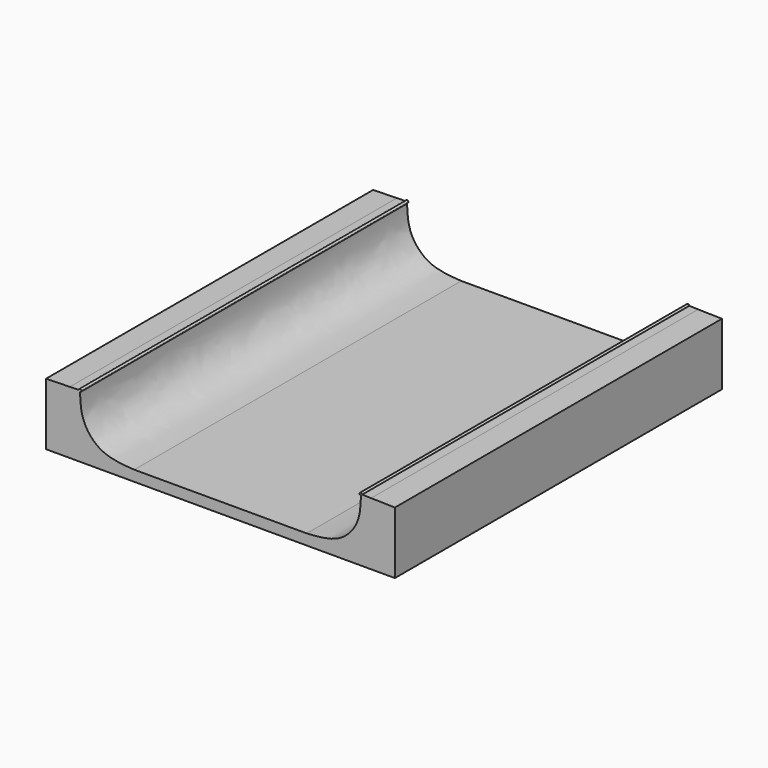
from build123d import *

# Parameters (mm, degrees)
F0_W     = 107.1716099977
F0_H     = 6.6367755644
F1_DEPTH = 254


# Not quite as in the source:
# - ends of sketch curves that miss each other by under 0.0002 mm in the source are joined


with BuildPart() as f1:
    # F0 (on Front) → F1 (new body)
    with BuildSketch(Plane.XZ):
        with BuildLine():
            Line((-53.5858049989, -3.3183877822), (-53.5858049989, 3.3183877822))
            add(Edge.make_bspline(
                [(-53.5858049989, 3.3183877822), (-60.7905189574, 3.7842082585), (-74.5629530695, 4.6746644037), (-86.6963968754, 19.2661575582), (-87.1229924092, 29.8680118762), (-87.2426380733, 34.9518884332)],
                knots=[0, 0, 0, 0, 0.3582791422, 0.6848815801, 0.984054993, 0.984054993, 0.984054993, 0.984054993], degree=3))
            ThreePointArc((-87.2426380733, 34.9518884332), (-87.8230310318, 35.1768908631), (-88.0742459033, 35.7464285425))
            Line((-88.0742459033, 35.7464285425), (-93.6096602081, 35.6210684855))
            Line((-93.6096602081, 35.6210684855), (-108.3679497242, 35.286838758))
            Line((-108.3679497242, 35.286838758), (-108.3679497242, -3.3183877822))
            Line((-108.3679497242, -3.3183877822), (-53.5858049989, -3.3183877822))
        make_face()
        with BuildLine():
            add(Edge.make_bspline(
                [(53.5858049989, 3.3183877822), (60.7905189574, 3.7842082585), (74.5629530695, 4.6746644037), (86.6963968754, 19.2661575582), (87.1229924092, 29.8680118762), (87.2426380733, 34.9518884332)],
                knots=[0, 0, 0, 0, 0.3582791422, 0.6848815801, 0.984054993, 0.984054993, 0.984054993, 0.984054993], degree=3))
            Line((53.5858049989, 3.3183877822), (53.5858049989, -3.3183877822))
            Line((53.5858049989, -3.3183877822), (108.3679497242, -3.3183877822))
            Line((108.3679497242, -3.3183877822), (108.3679497242, 35.286838758))
            Line((108.3679497242, 35.286838758), (93.6096602081, 35.6210684855))
            Line((93.6096602081, 35.6210684855), (88.0742459033, 35.7464285425))
            ThreePointArc((88.0742459033, 35.7464285425), (87.8230310318, 35.1768908631), (87.2426380733, 34.9518884332))
        make_face()
        Rectangle(F0_W, F0_H)
        with BuildLine():
            add(Edge.make_bspline(
                [(-87.2426380733, 34.9518884332), (-87.2490148129, 35.2228431489), (-87.2551520855, 35.4938413246), (-87.2612893581, 35.7648395002)],
                knots=[0.984054993, 0.984054993, 0.984054993, 0.984054993, 1, 1, 1, 1], degree=3))
            ThreePointArc((-87.2426380733, 34.9518884332), (-86.6797380364, 35.1964774959), (-86.448124364, 35.7648395002))
            ThreePointArc((-86.448124364, 35.7648395002), (-87.270495427, 36.5779523805), (-88.0742459033, 35.7464285425))
            Line((-88.0742459033, 35.7464285425), (-87.2612893581, 35.7648395002))
        make_face()
        with BuildLine():
            ThreePointArc((-88.0742459033, 35.7464285425), (-87.8230310318, 35.1768908631), (-87.2426380733, 34.9518884332))
            add(Edge.make_bspline(
                [(-87.2426380733, 34.9518884332), (-87.2490148129, 35.2228431489), (-87.2551520855, 35.4938413246), (-87.2612893581, 35.7648395002)],
                knots=[0.984054993, 0.984054993, 0.984054993, 0.984054993, 1, 1, 1, 1], degree=3))
            Line((-87.2612893581, 35.7648395002), (-88.0742459033, 35.7464285425))
        make_face()
        with BuildLine():
            add(Edge.make_bspline(
                [(87.2426380733, 34.9518884332), (87.2490148129, 35.2228431489), (87.2551520855, 35.4938413246), (87.2612893581, 35.7648395002)],
                knots=[0.984054993, 0.984054993, 0.984054993, 0.984054993, 1, 1, 1, 1], degree=3))
            ThreePointArc((87.2426380733, 34.9518884332), (87.8230310318, 35.1768908631), (88.0742459033, 35.7464285425))
            Line((88.0742459033, 35.7464285425), (87.2612893581, 35.7648395002))
        make_face()
        with BuildLine():
            ThreePointArc((88.0744543523, 35.7648395002), (86.6929273539, 36.346390822), (87.2426380733, 34.9518884332))
            add(Edge.make_bspline(
                [(87.2426380733, 34.9518884332), (87.2490148129, 35.2228431489), (87.2551520855, 35.4938413246), (87.2612893581, 35.7648395002)],
                knots=[0.984054993, 0.984054993, 0.984054993, 0.984054993, 1, 1, 1, 1], degree=3))
            Line((87.2612893581, 35.7648395002), (88.0742459033, 35.7464285425))
            ThreePointArc((88.0742459033, 35.7464285425), (88.0744022384, 35.7556334313), (88.0744543523, 35.7648395002))
        make_face()
    extrude(amount=F1_DEPTH)


solid = f1.part
